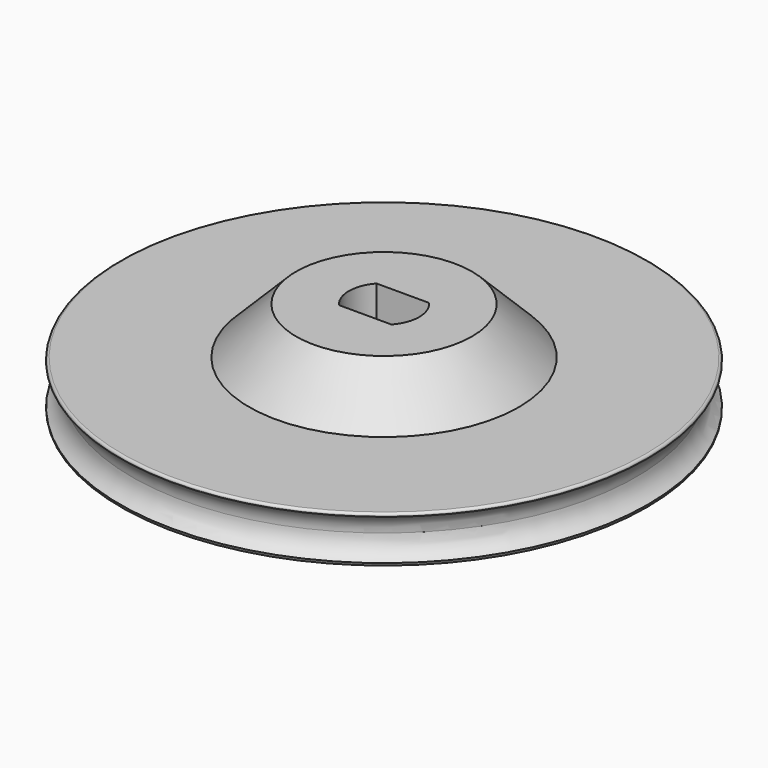
from build123d import *

# Parameters (mm, degrees)
F0_R     = 22.5
F1_DEPTH = 4
F2_R     = 2
F4_R     = 0.2
F5_R     = 12.5
F6_DEPTH = 4


# Not quite as in the source:
# - a fillet or chamfer that OpenCascade refuses, or shapes differently, is made with other operations: its cross-section is extruded or revolved along the edge and cut away or added


with BuildPart() as f1:
    # F0 (on Top) → F1 (new body)
    with BuildSketch(Plane.XY):
        Circle(F0_R)
        with BuildLine():
            ThreePointArc((2.2360679775, 2), (2.8025170769, 1.0704662693), (3, 0))
            ThreePointArc((3, 0), (2.8025170769, -1.0704662693), (2.2360679775, -2))
            ThreePointArc((2.2360679775, -2), (0, -3), (-2.2360679775, -2))
            ThreePointArc((-2.2360679775, -2), (-3, 0), (-2.2360679775, 2))
            ThreePointArc((-2.2360679775, 2), (0, 3), (2.2360679775, 2))
        make_face(mode=Mode.SUBTRACT)
        with BuildLine():
            ThreePointArc((-2.2360679775, -2), (0, -3), (2.2360679775, -2))
            Line((2.2360679775, -2), (-2.2360679775, -2))
        make_face()
        with BuildLine():
            Line((-2.2360679775, 2), (2.2360679775, 2))
            ThreePointArc((2.2360679775, 2), (0, 3), (-2.2360679775, 2))
        make_face()
    extrude(amount=F1_DEPTH)

    # F2 (on Front) → F3 (revolve, cut)
    with BuildSketch(Plane.XZ):
        with Locations((-23.5, 2)):
            Circle(F2_R)
    revolve(axis=Axis((0, 0, 4), (0, 0, 1)), mode=Mode.SUBTRACT)

    # F4
    f4_edges = [f1.edges().sort_by_distance(p)[0] for p in [
        (-22.5, 0, 4),
        (-22.5, 0, 0),
    ]]
    fillet(f4_edges, radius=F4_R)

    # F5 (on face) → F6 (join)
    with BuildSketch(Plane.XY.offset(4)):
        Circle(F5_R)
        with BuildLine():
            Line((2.2360679775, -2), (-2.2360679775, -2))
            ThreePointArc((-2.2360679775, -2), (-3, 0), (-2.2360679775, 2))
            Line((-2.2360679775, 2), (2.2360679775, 2))
            ThreePointArc((2.2360679775, 2), (3, 0), (2.2360679775, -2))
        make_face(mode=Mode.SUBTRACT)
    extrude(amount=F6_DEPTH)

    # F7: chamfer of 5 on 1 edges, made by hand


with BuildPart() as f7_tool2:
    # F7_s3 → F7_t4 (revolve)
    with BuildSketch(Plane.XZ):
        Polygon((7.5, 8), (12.5, 3), (12.5, 8), align=None)
    revolve(axis=Axis((0, 0, 8), (0, 0, 1)))

    split(bisect_by=Plane.XY.offset(4), keep=Keep.TOP)


with BuildPart() as f1_1:
    add(f1.part)

    # F7_t1: cut F7_tool2
    add(f7_tool2.part, mode=Mode.SUBTRACT)


solid = f1_1.part
